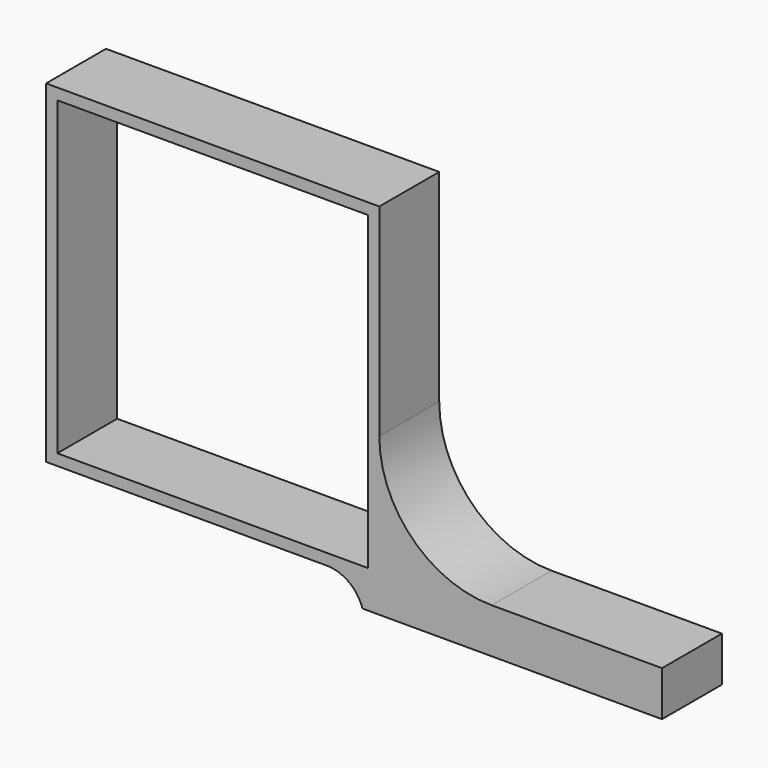
from build123d import *

# Parameters (mm, degrees)
F0_W        = 44.5
F0_H        = 44.5
F1_DEPTH    = 10
F2_W        = 41.5
F2_H        = 41.5
F3_DEPTH    = 10
F5_START    = 20
F4_W        = 10
F4_H        = 6
F5_DEPTH    = 40
F6_W        = 18.9917886164
F6_H        = 12.0773017406
F7_DEPTH    = 25
F8_R        = 15
F9_T1_DEPTH = 10


# Not quite as in the source:
# - a fillet or chamfer that OpenCascade refuses, or shapes differently, is made with other operations: its cross-section is extruded or revolved along the edge and cut away or added


with BuildPart() as f1:
    # F0 (on Front) → F1 (new body)
    with BuildSketch(Plane.XZ):
        Rectangle(F0_W, F0_H)
    extrude(amount=F1_DEPTH)

    # F2 (on Front) → F3 (cut)
    with BuildSketch(Plane.XZ):
        Rectangle(F2_W, F2_H)
    extrude(amount=F3_DEPTH, mode=Mode.SUBTRACT)

    # F4 (on Right) → F5 (join)
    with BuildSketch(Plane.YZ.offset(F5_START)):
        with Locations((-5, -22.75)):
            Rectangle(F4_W, F4_H)
    extrude(amount=F5_DEPTH)

    # F6 (on Front) → F7 (cut)
    with BuildSketch(Plane.XZ):
        with Locations((11.2541056918, -14.7113491297)):
            Rectangle(F6_W, F6_H)
    extrude(amount=F7_DEPTH, mode=Mode.SUBTRACT)

    # F8
    f8_edges = [f1.edges().sort_by_distance(p)[0] for p in [
        (22.25, -5, -19.75),
    ]]
    fillet(f8_edges, radius=F8_R)

    # F9: fillet of radius 5 on 1 edges, made by hand

    # F9_s2 → F9_t1 (join)
    with BuildSketch(Plane.XZ):
        with BuildLine():
            ThreePointArc((20, -25.75), (18.1883438845, -23.2188711259), (15.2303039929, -22.25))
            Line((15.2303039929, -22.25), (20, -22.25))
            Line((20, -22.25), (20, -25.75))
        make_face()
    extrude(amount=F9_T1_DEPTH)


solid = f1.part
